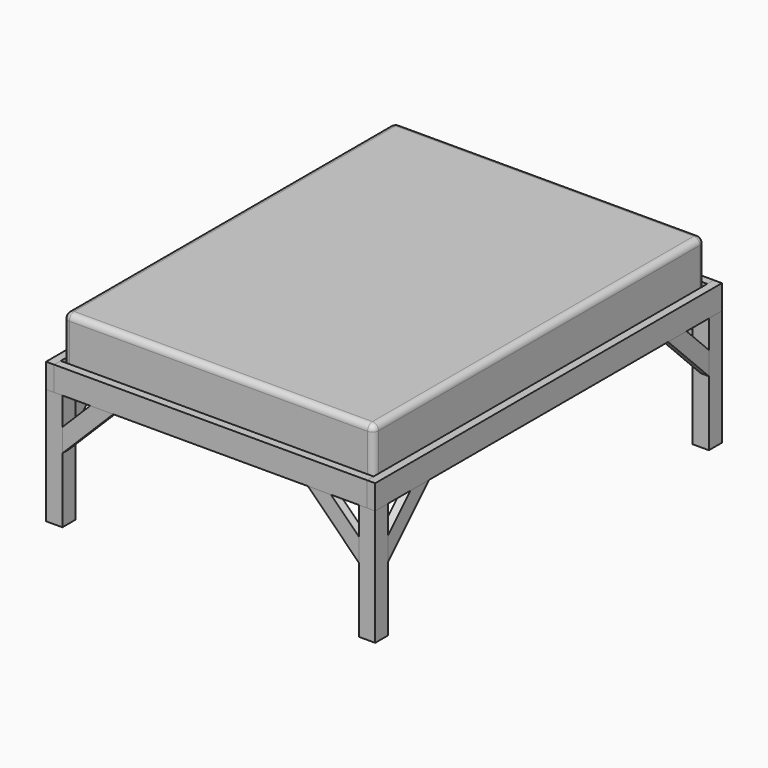
from build123d import *

# Parameters (mm, degrees)
F1_W      = 1524
F1_H      = 2032
F2_DEPTH  = 250
F3_R      = 30
F5_DEPTH  = 80
F4_W      = 1536
F4_H      = 40
F6_DEPTH  = 80
F4_W_2    = 1524
F7_DEPTH  = 40
F8_DEPTH  = 40
F9_DEPTH  = 40
F10_DEPTH = 40
F11_W     = 80
F11_H     = 80
F13_DEPTH = 570
F11_W_2   = 40
F15_DEPTH = 40
F17_DEPTH = 40
F19_DEPTH = 40
F21_DEPTH = 40


with BuildPart() as f2:
    # F1 (on Top) → F2 (new body)
    with BuildSketch(Plane.XY):
        Rectangle(F1_W, F1_H)
    extrude(amount=F2_DEPTH)

    # F3
    f3_edges = [f2.edges().sort_by_distance(p)[0] for p in [
        (-762, 0, 250),
        (0, 1016, 250),
        (762, 0, 250),
        (0, -1016, 250),
        (-762, -1016, 125),
        (-762, 1016, 125),
        (762, -1016, 125),
        (0, -1016, 0),
        (-762, 0, 0),
        (762, 1016, 125),
        (762, 0, 0),
        (0, 1016, 0),
    ]]
    fillet(f3_edges, radius=F3_R)


with BuildPart() as f5:
    # F4 (on face) → F5 (new body)
    with BuildSketch(Plane.XY):
        Polygon((-768, 840), (-768, 1024), (-768, 1064), (-808, 1064), (-808, -1064), (-768, -1064), (-768, -1024), (-768, -840), (-768, -800), (-768, -430), (-768, -390), (-768, -20), (-768, 20), (-768, 390), (-768, 430), (-768, 800), align=None)
    extrude(amount=-F5_DEPTH)

    # F4 (on face) → F9 (join)
    with BuildSketch(Plane.XY):
        Polygon((-768, 840), (-768, 1024), (-768, 1064), (-808, 1064), (-808, -1064), (-768, -1064), (-768, -1024), (-768, -840), (-768, -800), (-768, -430), (-768, -390), (-768, -20), (-768, 20), (-768, 390), (-768, 430), (-768, 800), align=None)
    extrude(amount=F9_DEPTH)


with BuildPart() as f5b:
    # F4 (on face) → F5, piece 2 (new body)
    with BuildSketch(Plane.XY):
        Polygon((768, 1064), (768, 1024), (768, 840), (768, 800), (768, 430), (768, 390), (768, 20), (768, -20), (768, -390), (768, -430), (768, -800), (768, -840), (768, -1024), (768, -1064), (808, -1064), (808, 1064), align=None)
    extrude(amount=-F5_DEPTH)

    # F4 (on face) → F7 (join)
    with BuildSketch(Plane.XY):
        Polygon((768, 1064), (768, 1024), (768, 840), (768, 800), (768, 430), (768, 390), (768, 20), (768, -20), (768, -390), (768, -430), (768, -800), (768, -840), (768, -1024), (768, -1064), (808, -1064), (808, 1064), align=None)
    extrude(amount=F7_DEPTH)


with BuildPart() as f6:
    # F4 (on face) → F6 (new body)
    with BuildSketch(Plane.XY):
        with Locations((0, 1044)):
            Rectangle(F4_W, F4_H)
    extrude(amount=-F6_DEPTH)

    # F4 (on face) → F8 (join)
    with BuildSketch(Plane.XY):
        with Locations((0, 1044)):
            Rectangle(F4_W, F4_H)
    extrude(amount=F8_DEPTH)


with BuildPart() as f6b:
    # F4 (on face) → F6, piece 2 (new body)
    with BuildSketch(Plane.XY):
        with Locations((0, 820)):
            Rectangle(F4_W_2, F4_H)
    extrude(amount=-F6_DEPTH)


with BuildPart() as f6c:
    # F4 (on face) → F6, piece 3 (new body)
    with BuildSketch(Plane.XY):
        with Locations((0, 410)):
            Rectangle(F4_W_2, F4_H)
    extrude(amount=-F6_DEPTH)


with BuildPart() as f6d:
    # F4 (on face) → F6, piece 4 (new body)
    with BuildSketch(Plane.XY):
        Rectangle(F4_W_2, F4_H)
    extrude(amount=-F6_DEPTH)


with BuildPart() as f6e:
    # F4 (on face) → F6, piece 5 (new body)
    with BuildSketch(Plane.XY):
        with Locations((0, -410)):
            Rectangle(F4_W_2, F4_H)
    extrude(amount=-F6_DEPTH)


with BuildPart() as f6f:
    # F4 (on face) → F6, piece 6 (new body)
    with BuildSketch(Plane.XY):
        with Locations((0, -820)):
            Rectangle(F4_W_2, F4_H)
    extrude(amount=-F6_DEPTH)


with BuildPart() as f6g:
    # F4 (on face) → F6, piece 7 (new body)
    with BuildSketch(Plane.XY):
        with Locations((0, -1044)):
            Rectangle(F4_W, F4_H)
    extrude(amount=-F6_DEPTH)

    # F4 (on face) → F10 (join)
    with BuildSketch(Plane.XY):
        with Locations((0, -1044)):
            Rectangle(F4_W, F4_H)
    extrude(amount=F10_DEPTH)


with BuildPart() as f13:
    # F11 (on face) → F13 (new body, through all)
    with BuildSketch(Plane(origin=(0, 0, -80), x_dir=(1, 0, 0), z_dir=(0, 0, -1))):
        with Locations((-768, 1024)):
            Rectangle(F11_W, F11_H)
    extrude(amount=F13_DEPTH)


with BuildPart() as f13b:
    # F11 (on face) → F13, piece 2 (new body, through all)
    with BuildSketch(Plane(origin=(0, 0, -80), x_dir=(1, 0, 0), z_dir=(0, 0, -1))):
        with Locations((788, 1024)):
            Rectangle(F11_W_2, F11_H)
        with Locations((748, 1024)):
            Rectangle(F11_W_2, F11_H)
    extrude(amount=F13_DEPTH)


with BuildPart() as f13c:
    # F11 (on face) → F13, piece 3 (new body, through all)
    with BuildSketch(Plane(origin=(0, 0, -80), x_dir=(1, 0, 0), z_dir=(0, 0, -1))):
        with Locations((788, -1024)):
            Rectangle(F11_W_2, F11_H)
        with Locations((748, -1024)):
            Rectangle(F11_W_2, F11_H)
    extrude(amount=F13_DEPTH)


with BuildPart() as f13d:
    # F11 (on face) → F13, piece 4 (new body, through all)
    with BuildSketch(Plane(origin=(0, 0, -80), x_dir=(1, 0, 0), z_dir=(0, 0, -1))):
        with Locations((-768, -1024)):
            Rectangle(F11_W, F11_H)
    extrude(amount=F13_DEPTH)


with BuildPart() as f15:
    # F14 (on face) → F15 (new body, through all)
    with BuildSketch(Plane.XZ.offset(1064)):
        Polygon((-728, -216.8629150101), (-728, -330), (-478, -80), (-591.1370849899, -80), align=None)
    extrude(amount=-F15_DEPTH)


with BuildPart() as f15b:
    # F14 (on face) → F15, piece 2 (new body, through all)
    with BuildSketch(Plane.XZ.offset(1064)):
        Polygon((591.1370849899, -80), (478, -80), (728, -330), (728, -216.8629150101), align=None)
    extrude(amount=-F15_DEPTH)


with BuildPart() as f17:
    # F16 (on face) → F17 (new body, through all)
    with BuildSketch(Plane(origin=(0, 1064, 0), x_dir=(-1, 0, 0), z_dir=(0, 1, 0))):
        Polygon((-591.1370849898, -80), (-728, -216.8629150102), (-728, -330), (-478, -80), align=None)
    extrude(amount=-F17_DEPTH)


with BuildPart() as f17b:
    # F16 (on face) → F17, piece 2 (new body, through all)
    with BuildSketch(Plane(origin=(0, 1064, 0), x_dir=(-1, 0, 0), z_dir=(0, 1, 0))):
        Polygon((591.1370849899, -80), (478, -80), (728, -330), (728, -216.8629150102), align=None)
    extrude(amount=-F17_DEPTH)


with BuildPart() as f19:
    # F18 (on face) → F19 (new body, through all)
    with BuildSketch(Plane.YZ.offset(808)):
        Polygon((-984, -330), (-734, -80), (-847.1370849899, -80), (-984, -216.8629150101), align=None)
    extrude(amount=-F19_DEPTH)


with BuildPart() as f19b:
    # F18 (on face) → F19, piece 2 (new body, through all)
    with BuildSketch(Plane.YZ.offset(808)):
        Polygon((734, -80), (984, -330), (984, -216.8629150101), (847.1370849899, -80), align=None)
    extrude(amount=-F19_DEPTH)


with BuildPart() as f21:
    # F20 (on face) → F21 (new body, through all)
    with BuildSketch(Plane(origin=(-808, 0, 0), x_dir=(0, -1, 0), z_dir=(-1, 0, 0))):
        Polygon((-847.1370849899, -80), (-984, -216.8629150101), (-984, -330), (-734, -80), align=None)
    extrude(amount=-F21_DEPTH)


with BuildPart() as f21b:
    # F20 (on face) → F21, piece 2 (new body, through all)
    with BuildSketch(Plane(origin=(-808, 0, 0), x_dir=(0, -1, 0), z_dir=(-1, 0, 0))):
        Polygon((984, -216.8629150101), (847.1370849899, -80), (734, -80), (984, -330), align=None)
    extrude(amount=-F21_DEPTH)


solid = Compound([f2.part, f5.part, f5b.part, f6.part, f6b.part, f6c.part, f6d.part, f6e.part, f6f.part, f6g.part, f13.part, f13b.part, f13c.part, f13d.part, f15.part, f15b.part, f17.part, f17b.part, f19.part, f19b.part, f21.part, f21b.part])
